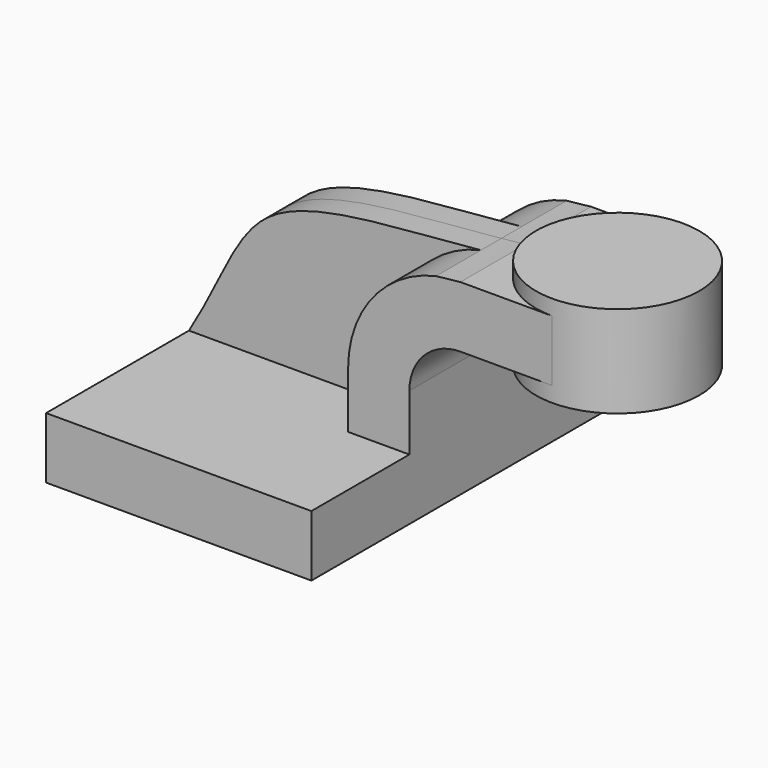
from build123d import *

# Parameters (mm, degrees)
F1_DEPTH = 63.5
F2_DEPTH = 25.4
F3_DEPTH = 7.9375
F0_W     = 25.4
F0_H     = 19.05
F4_DEPTH = 25.4


# Not quite as in the source:
# - a feature names something its author has since deleted; it is built from what else it names


with BuildPart() as f1:
    # F0 (on Front) → F1 (new body, symmetric)
    with BuildSketch(Plane.XZ):
        Polygon((-41.275, 9.525), (-41.275, -9.525), (41.275, -9.525), (41.275, 9.525), (22.225, 9.525), align=None)
    extrude(amount=F1_DEPTH, both=True)

    # F0 (on Front) → F2 (join, symmetric)
    with BuildSketch(Plane.XZ):
        with BuildLine():
            Line((22.225, 9.525), (41.275, 9.525))
            Line((41.275, 9.525), (41.275, 27.0002))
            ThreePointArc((41.275, 27.0002), (45.9246798487, 38.2255201513), (57.15, 42.8752))
            Line((57.15, 42.8752), (60.325, 42.8752))
            Line((60.325, 42.8752), (60.325, 61.9252))
            Line((60.325, 61.9252), (57.15, 61.9252))
            add(Edge.make_bspline(
                [(49.5546191044, 61.0892864361), (52.0673413898, 61.343380394), (54.6014869269, 61.6190974593), (57.15, 61.9252)],
                knots=[0.9527141081, 0.9527141081, 0.9527141081, 0.9527141081, 1, 1, 1, 1], degree=3))
            ThreePointArc((49.5546191044, 61.0892864361), (29.9009238434, 48.8461029022), (22.225, 27.0002))
            Line((22.225, 27.0002), (22.225, 9.525))
        make_face()
    extrude(amount=F2_DEPTH, both=True)

    # F0 (on Front) → F3 (join, symmetric)
    with BuildSketch(Plane.XZ):
        with BuildLine():
            add(Edge.make_bspline(
                [(-41.275, 9.525), (-30.0133153796, 28.1962957233), (-23.3223965861, 57.9111150093), (22.6888247137, 58.3725373278), (49.5546191044, 61.0892864361)],
                knots=[0, 0, 0, 0, 0.4471377236, 0.9527141081, 0.9527141081, 0.9527141081, 0.9527141081], degree=3))
            Line((-41.275, 9.525), (22.225, 9.525))
            Line((22.225, 9.525), (22.225, 27.0002))
            ThreePointArc((22.225, 27.0002), (29.9009238434, 48.8461029022), (49.5546191044, 61.0892864361))
        make_face()
    extrude(amount=F3_DEPTH, both=True)

    # F0 (on Front) → F4 (join, symmetric)
    with BuildSketch(Plane.XZ):
        with Locations((73.025, 52.4002)):
            Rectangle(F0_W, F0_H)
    extrude(amount=F4_DEPTH, both=True)

    # F0 (on Front) → F5 (revolve)
    with BuildSketch(Plane.XZ):
        Polygon((85.725, 66.675), (85.725, 61.9252), (85.725, 42.8752), (85.725, 38.1), (111.125, 38.1), (111.125, 66.675), align=None)
    revolve(axis=Axis((85.725, 0, 52.3875), (0, 0, -1)))


solid = f1.part
